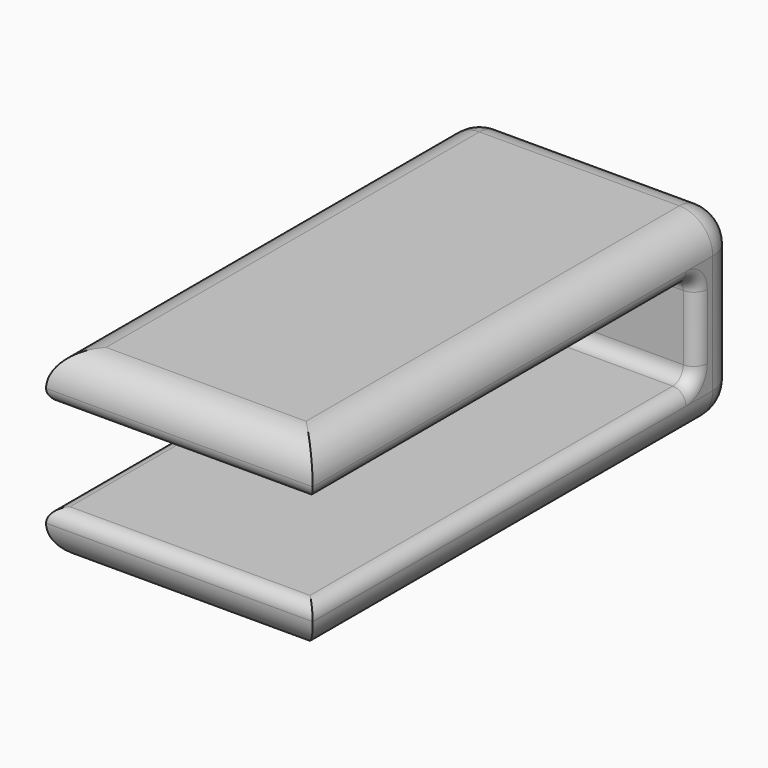
from build123d import *

# Parameters (mm, degrees)
F0_W     = 10
F0_H     = 18
F1_DEPTH = 1.75
F2_W     = 10
F2_H     = 1.75
F2_H_2   = 5.2
F3_DEPTH = 2
F8_R     = 0.5
F9_R     = 1.24999


# Not quite as in the source:
# - a fillet or chamfer is up to 0.001 mm smaller than in the source, because OpenCascade refuses the exact size


with BuildPart() as f1:
    # F0 (on Top) → F1 (new body)
    with BuildSketch(Plane.XY):
        Rectangle(F0_W, F0_H)
    extrude(amount=F1_DEPTH)

    # F2 (on face) → F3 (join)
    with BuildSketch(Plane(origin=(0, 9, 0), x_dir=(-1, 0, 0), z_dir=(0, 1, 0))):
        with Locations((0, 0.875)):
            Rectangle(F2_W, F2_H)
        with Locations((0, -2.6)):
            Rectangle(F2_W, F2_H_2)
    extrude(amount=F3_DEPTH)

    # F7: F1 across plane


with BuildPart() as f1_1:
    add(f1.part)
    add(f1.part.mirror(Plane(origin=(-5, 1.2789499015, -1.725), x_dir=(0.9979743188, 0.063618071, 0), z_dir=(0, 0, -1))))

    # F8
    f8_edges = [f1_1.edges().sort_by_distance(p)[0] for p in [
        (0, 9, 0),
        (0, 9, -3.45),
        (5, 0, -3.45),
        (-5, 0, -3.45),
        (0, -9, -3.45),
        (5, 0, 0),
        (-5, 0, 0),
        (0, -9, 0),
        (5, 9, -1.725),
        (-5, 9, -1.725),
    ]]
    fillet(f8_edges, radius=F8_R)

    # F9 (radius 1.25 in the source; OpenCascade refuses exactly that, so slightly less here)
    f9_edges = [f1_1.edges().sort_by_distance(p)[0] for p in [
        (5, 11, -1.725),
        (0, 11, -5.2),
        (-5, 11, -1.725),
        (0, 11, 1.75),
        (5, 1, 1.75),
        (-5, 1, 1.75),
        (0, -9, 1.75),
        (-5, 1, -5.2),
        (0, -9, -5.2),
        (5, 1, -5.2),
    ]]
    fillet(f9_edges, radius=F9_R)


solid = f1_1.part
